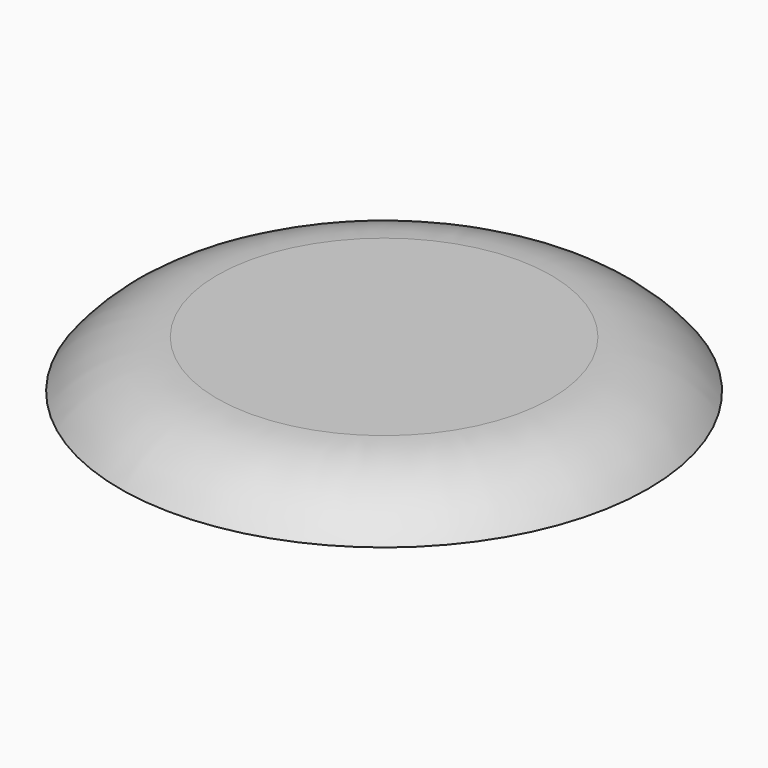
from build123d import *

# Parameters (mm, degrees)
F0_R     = 11
F2_DEPTH = 2
F1_R     = 3.175
F3_DEPTH = 3


# Not quite as in the source:
# - a fillet or chamfer that OpenCascade refuses, or shapes differently, is made with other operations: its cross-section is extruded or revolved along the edge and cut away or added


with BuildPart() as f2:
    # F0 (on Top) → F2 (new body)
    with BuildSketch(Plane.XY):
        Circle(F0_R)
    extrude(amount=F2_DEPTH)

    # F1 (on Top) → F3 (join)
    with BuildSketch(Plane.XY):
        Circle(F1_R)
    extrude(amount=-F3_DEPTH)

    # F4: fillet of radius 5.08 on 1 edges, made by hand

    # F4_s1 → F4_t2 (revolve, cut)
    with BuildSketch(Plane.XZ):
        with BuildLine():
            ThreePointArc((11, 0), (9.2140835586, 1.4726256161), (6.9601980247, 2))
            Line((6.9601980247, 2), (11, 2))
            Line((11, 2), (11, 0))
        make_face()
    revolve(axis=Axis((0, 0, 2), (0, 0, 1)), mode=Mode.SUBTRACT)


solid = f2.part
